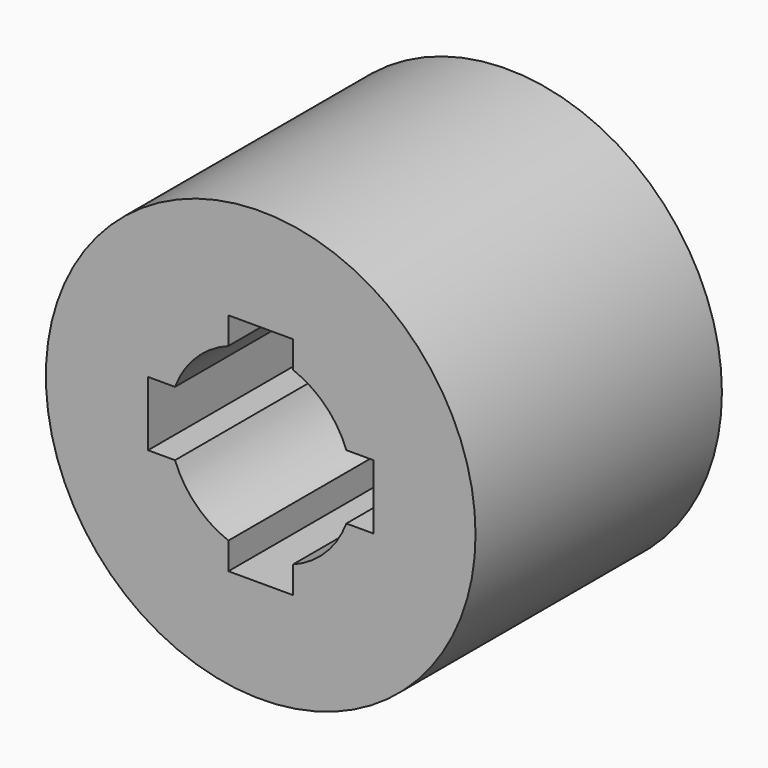
from build123d import *

# Parameters (mm, degrees)
F0_R     = 4.06
F1_DEPTH = 5.82
F3_DEPTH = 4.06
F4_R     = 1.18
F5_DEPTH = 25
F6_R     = 2.5
F6_R_2   = 1.18
F7_DEPTH = 1.6


# Not quite as in the source:
# - a feature names something its author has since deleted; it is built from what else it names


with BuildPart() as f1:
    # F0 (on Front) → F1 (new body)
    with BuildSketch(Plane.XZ):
        Circle(F0_R)
    extrude(amount=F1_DEPTH)

    # F2 (on face) → F3 (cut)
    with BuildSketch(Plane.XZ.offset(5.82)):
        with BuildLine():
            ThreePointArc((1.6188885076, -0.61), (1.7019954639, -0.3100184526), (1.73, 0))
            ThreePointArc((1.73, 0), (1.7019954639, 0.3100184526), (1.6188885076, 0.61))
            ThreePointArc((1.6188885076, 0.61), (1.2232947315, 1.2232947315), (0.61, 1.6188885076))
            ThreePointArc((0.61, 1.6188885076), (0, 1.73), (-0.61, 1.6188885076))
            ThreePointArc((-0.61, 1.6188885076), (-1.2232947315, 1.2232947315), (-1.6188885076, 0.61))
            ThreePointArc((-1.6188885076, 0.61), (-1.73, 0), (-1.6188885076, -0.61))
            ThreePointArc((-1.6188885076, -0.61), (-1.2232947315, -1.2232947315), (-0.61, -1.6188885076))
            ThreePointArc((-0.61, -1.6188885076), (0, -1.73), (0.61, -1.6188885076))
            ThreePointArc((0.61, -1.6188885076), (1.2232947315, -1.2232947315), (1.6188885076, -0.61))
        make_face()
        with BuildLine():
            ThreePointArc((1.6188885076, 0.61), (1.7019954639, 0.3100184526), (1.73, 0))
            ThreePointArc((1.73, 0), (1.7019954639, -0.3100184526), (1.6188885076, -0.61))
            Line((1.6188885076, -0.61), (2.1288885076, -0.61))
            Line((2.1288885076, -0.61), (2.1288885076, 0.61))
            Line((2.1288885076, 0.61), (1.6188885076, 0.61))
        make_face()
        with BuildLine():
            ThreePointArc((-0.61, 1.6188885076), (0, 1.73), (0.61, 1.6188885076))
            Line((0.61, 1.6188885076), (0.61, 2.1288885076))
            Line((0.61, 2.1288885076), (-0.61, 2.1288885076))
            Line((-0.61, 2.1288885076), (-0.61, 1.6188885076))
        make_face()
        with BuildLine():
            Line((0.61, -2.1288885076), (0.61, -1.6188885076))
            ThreePointArc((0.61, -1.6188885076), (0, -1.73), (-0.61, -1.6188885076))
            Line((-0.61, -1.6188885076), (-0.61, -2.1288885076))
            Line((-0.61, -2.1288885076), (0.61, -2.1288885076))
        make_face()
        with BuildLine():
            ThreePointArc((-1.6188885076, -0.61), (-1.73, 0), (-1.6188885076, 0.61))
            Line((-1.6188885076, 0.61), (-2.1288885076, 0.61))
            Line((-2.1288885076, 0.61), (-2.1288885076, -0.61))
            Line((-2.1288885076, -0.61), (-1.6188885076, -0.61))
        make_face()
    extrude(amount=-F3_DEPTH, mode=Mode.SUBTRACT)

    # F4 (on face) → F5 (cut)
    with BuildSketch(Plane.XZ.offset(1.76)):
        Circle(F4_R)
    extrude(amount=-F5_DEPTH, mode=Mode.SUBTRACT)

    # F6 (on face) → F7 (cut)
    with BuildSketch(Plane(origin=(0, 0, 0), x_dir=(-1, 0, 0), z_dir=(0, 1, 0))):
        Circle(F6_R)
        Circle(F6_R_2, mode=Mode.SUBTRACT)
    extrude(amount=-F7_DEPTH, mode=Mode.SUBTRACT)


solid = f1.part
